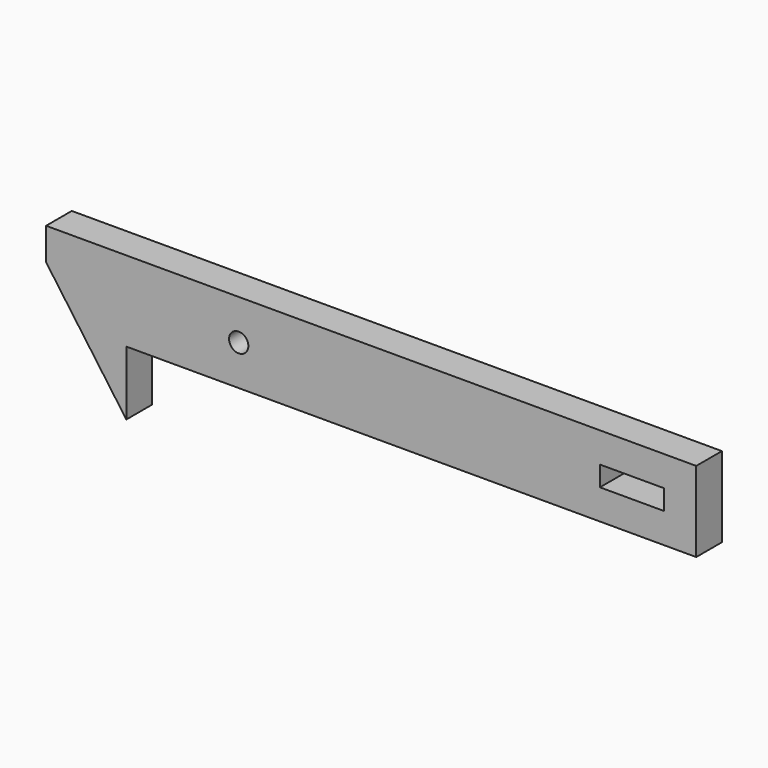
from build123d import *

# Parameters (mm, degrees)
F0_W     = 40.5
F0_H     = 5
F1_DEPTH = 2
F2_W     = 5
F2_H     = 4
F3_DEPTH = 2
F4_SIZE2 = 6.99999
F4_SIZE  = 4.99999
F5_W     = 4
F5_H     = 1.25
F6_DEPTH = 2
F7_R     = 0.6
F8_DEPTH = 2


# Not quite as in the source:
# - a fillet or chamfer is up to 0.001 mm smaller than in the source, because OpenCascade refuses the exact size


with BuildPart() as f1:
    # F0 (on Front) → F1 (new body)
    with BuildSketch(Plane.XZ):
        with Locations((-20.25, 2.5)):
            Rectangle(F0_W, F0_H)
    extrude(amount=F1_DEPTH)

    # F2 (on Front) → F3 (join)
    with BuildSketch(Plane.XZ):
        with Locations((-38, -2)):
            Rectangle(F2_W, F2_H)
    extrude(amount=F3_DEPTH)

    # F4 (size 5 and 7 in the source; OpenCascade refuses exactly that, so slightly less here)
    f4_edges = [f1.edges().sort_by_distance(p)[0] for p in [
        (-40.5, -1, -4),
    ]]
    f4_side = f1.faces().sort_by_distance((-38, -1, -4))[0]
    chamfer(f4_edges, length=F4_SIZE, length2=F4_SIZE2, reference=f4_side)

    # F5 (on face) → F6 (cut)
    with BuildSketch(Plane.XZ.offset(2)):
        with Locations((-4, 2.5)):
            Rectangle(F5_W, F5_H)
    extrude(amount=-F6_DEPTH, mode=Mode.SUBTRACT)

    # F7 (on face) → F8 (cut)
    with BuildSketch(Plane.XZ.offset(2)):
        with Locations((-28.5, 2.5)):
            Circle(F7_R)
    extrude(amount=-F8_DEPTH, mode=Mode.SUBTRACT)


solid = f1.part
